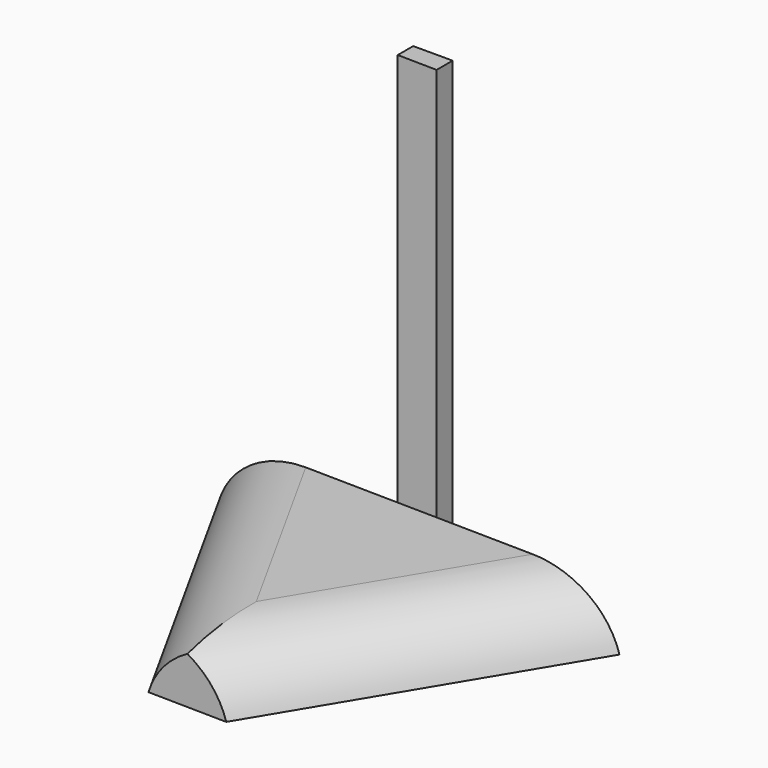
from build123d import *

# Parameters (mm, degrees)
F1_DEPTH      = 3.81
F2_SIZE       = 5.08
F3_T1_DEPTH   = 45.7068968586
F3_T3_DEPTH   = 45.7068968586
F5_DEPTH      = 25.4
F5_DEPTH_BACK = 3.81


# Not quite as in the source:
# - a fillet or chamfer that OpenCascade refuses, or shapes differently, is made with other operations: its cross-section is extruded or revolved along the edge and cut away or added


with BuildPart() as f1:
    # F0 (on Top) → F1 (new body)
    with BuildSketch(Plane.XY):
        Polygon((-0.2622354642, -15.1205231096), (13.2258748636, 7.3331589811), (-12.9636393994, 7.7873641286), align=None)
    extrude(amount=F1_DEPTH)

    # F2
    f2_edges = [f1.edges().sort_by_distance(p)[0] for p in [
        (-0.262235, -15.120523, 1.905),
    ]]
    chamfer(f2_edges, length=F2_SIZE)

    # F3: fillet of radius 5.08 on 2 edges, made by hand

    # F3_s2 → F3_t1 (cut)
    with BuildSketch(Plane(origin=(-10.4602488885, -17.4131955793, 0), x_dir=(0, 0, 1), z_dir=(0.5149420555, 0.8572249877, 0))):
        with BuildLine():
            ThreePointArc((0, 7.5613984578), (2.7460926284, 5.7535615814), (3.81, 2.6427096081))
            Line((3.81, 2.6427096081), (3.81, 7.5613984578))
            Line((3.81, 7.5613984578), (0, 7.5613984578))
        make_face()
    extrude(amount=F3_T1_DEPTH, mode=Mode.SUBTRACT)

    # F3_s4 → F3_t3 (cut)
    with BuildSketch(Plane(origin=(-12.3134758372, 22.2082312655, 0), x_dir=(0, 0, 1), z_dir=(0.4849075883, -0.8745653954, 0))):
        with BuildLine():
            ThreePointArc((3.81, 2.6427096081), (2.7460926284, 5.7535615814), (0, 7.5613984578))
            Line((0, 7.5613984578), (3.81, 7.5613984578))
            Line((3.81, 7.5613984578), (3.81, 2.6427096081))
        make_face()
    extrude(amount=F3_T3_DEPTH, mode=Mode.SUBTRACT)

    # F4 (on face) → F5 (join, two sides)
    with BuildSketch(Plane.XY.offset(3.81)) as f5_sk:
        Polygon((1.27, 7.5405099022), (1.27, 8.8325355317), (-1.27, 8.8325355317), (-1.27, 7.5845611611), align=None)
    extrude(amount=F5_DEPTH)
    extrude(f5_sk.sketch, amount=-F5_DEPTH_BACK)


solid = f1.part
